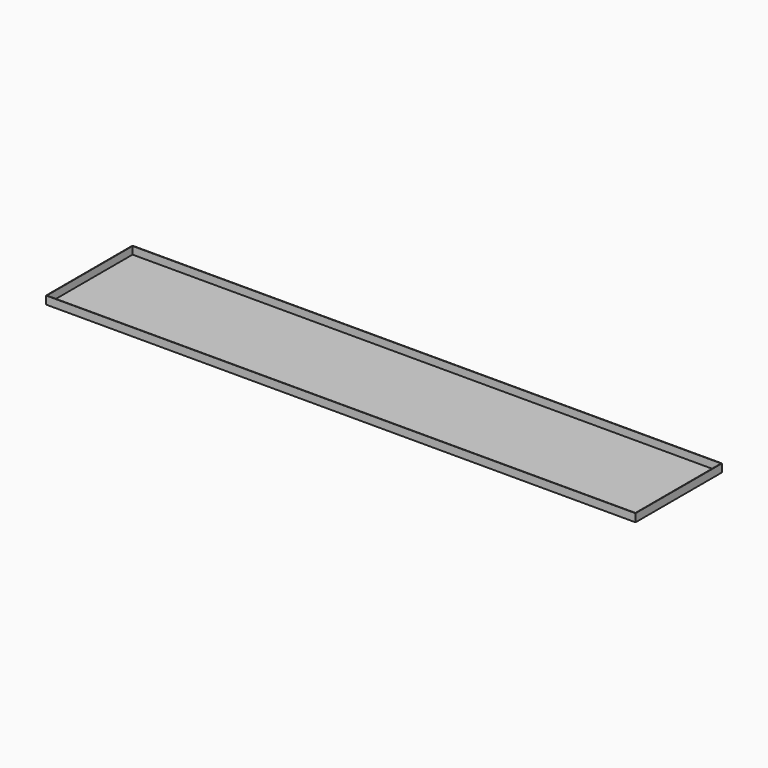
from build123d import *

# Parameters (mm, degrees)
F0_W     = 3743.325
F0_H     = 685.8
F0_W_2   = 3740.277
F0_H_2   = 682.752
F1_DEPTH = 50.8
F3_T     = -2.54


# Not quite as in the source:
# - the program builds the solid bodies; features that only make, move or delete a surface that nothing else refers to are left out


with BuildPart() as f1:
    # F0 (on Top) → F1 (new body)
    with BuildSketch(Plane.XY):
        with Locations((-1806.9549600244, 334.3743443951)):
            Rectangle(F0_W, F0_H)
        with Locations((-1806.9549600244, 334.3743443951)):
            Rectangle(F0_W_2, F0_H_2, mode=Mode.SUBTRACT)
        with Locations((-1806.9549600244, 334.3743443951)):
            Rectangle(F0_W_2, F0_H_2)
    extrude(amount=F1_DEPTH)

    # F3
    f3_openings = [f1.faces().sort_by_distance(p)[0] for p in [
        (-1806.95496, 334.374344, 50.8),
    ]]
    offset(amount=F3_T, openings=f3_openings)


solid = f1.part
